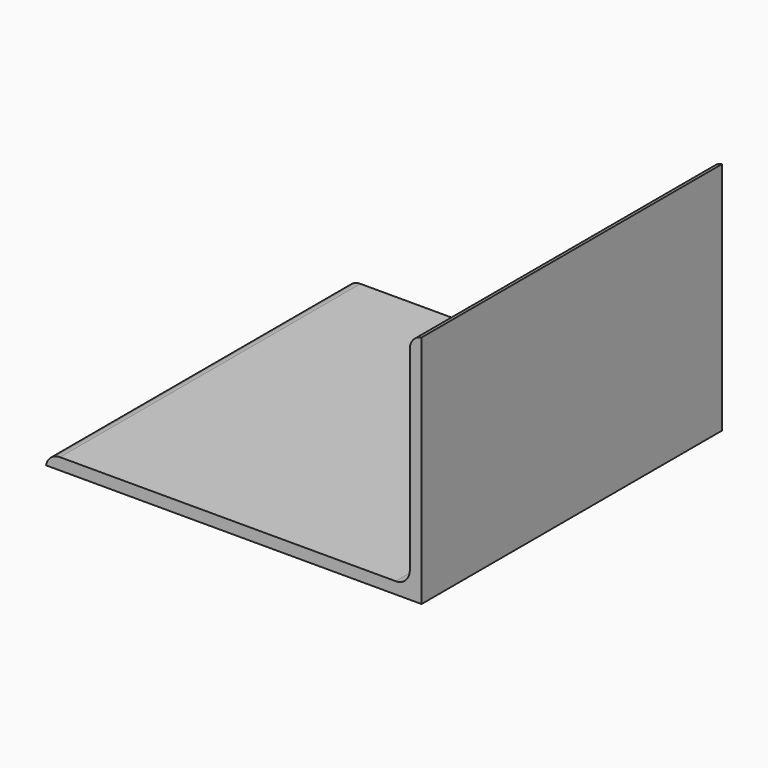
from build123d import *

# Parameters (mm, degrees)
F1_DEPTH    = 203.2
F2_T1_DEPTH = 203.2
F2_T3_DEPTH = 240.7671066227
F2_T5_DEPTH = 240.7671066227


# Not quite as in the source:
# - a fillet or chamfer that OpenCascade refuses, or shapes differently, is made with other operations: its cross-section is extruded or revolved along the edge and cut away or added


with BuildPart() as f1:
    # F0 (on Front) → F1 (new body)
    with BuildSketch(Plane.XZ):
        Polygon((-203.2, 0), (0, 0), (0, 127), (-6.35, 127), (-6.35, 6.35), (-203.2, 6.35), align=None)
    extrude(amount=F1_DEPTH)

    # F2: fillet of radius 7.62 on 3 edges, made by hand

    # F2_s2 → F2_t1 (join)
    with BuildSketch(Plane.XZ):
        with BuildLine():
            ThreePointArc((-13.97, 6.35), (-8.5818463274, 8.5818463274), (-6.35, 13.97))
            Line((-6.35, 13.97), (-6.35, 6.35))
            Line((-6.35, 6.35), (-13.97, 6.35))
        make_face()
    extrude(amount=F2_T1_DEPTH)

    # F2_s4 → F2_t3 (cut)
    with BuildSketch(Plane.XZ.offset(-18.7835533113)):
        with BuildLine():
            ThreePointArc((-195.6865786755, 6.35), (-200.6052675251, 4.5498711326), (-203.2, 0))
            Line((-203.2, 0), (-203.2, 6.35))
            Line((-203.2, 6.35), (-195.6865786755, 6.35))
        make_face()
    extrude(amount=F2_T3_DEPTH, mode=Mode.SUBTRACT)

    # F2_s6 → F2_t5 (cut)
    with BuildSketch(Plane.XZ.offset(-18.7835533113)):
        with BuildLine():
            ThreePointArc((-6.35, 119.4865786755), (-4.5498711326, 124.4052675251), (0, 127))
            Line((0, 127), (-6.35, 127))
            Line((-6.35, 127), (-6.35, 119.4865786755))
        make_face()
    extrude(amount=F2_T5_DEPTH, mode=Mode.SUBTRACT)


solid = f1.part
